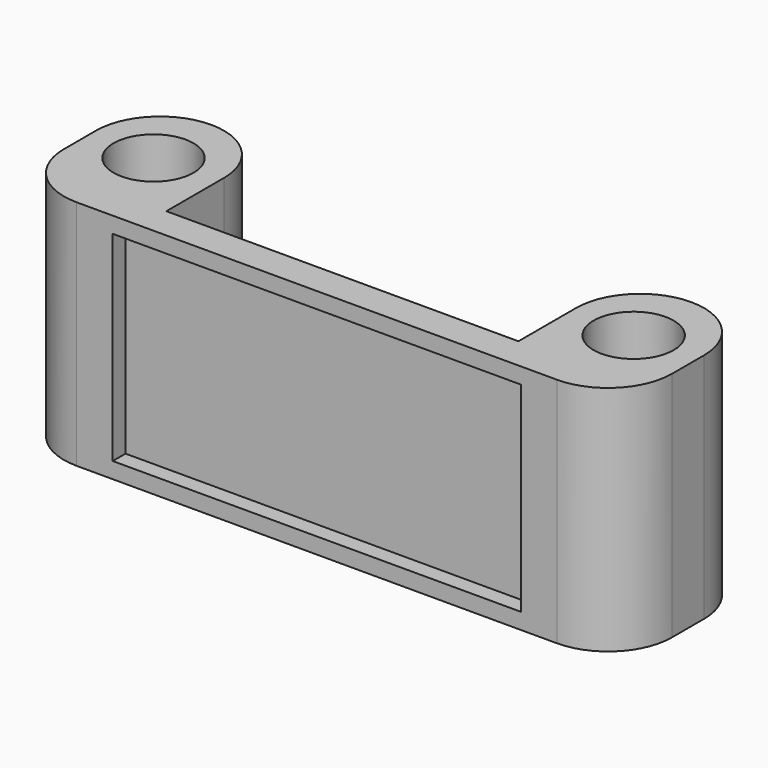
from build123d import *

# Parameters (mm, degrees)
F0_W     = 38
F0_H     = 14.5
F1_DEPTH = 2
F2_W     = 25.5
F2_H     = 12.5
F3_DEPTH = 1
F4_W     = 8
F4_H     = 14.5
F5_DEPTH = 8.5
F6_R     = 2.5
F7_DEPTH = 25
F9_DEPTH = 5
F10_R    = 3.99999


# Not quite as in the source:
# - a fillet or chamfer is up to 0.001 mm smaller than in the source, because OpenCascade refuses the exact size


with BuildPart() as f1:
    # F0 (on Front) → F1 (new body)
    with BuildSketch(Plane.XZ):
        Rectangle(F0_W, F0_H)
    extrude(amount=F1_DEPTH)

    # F2 (on face) → F3 (cut)
    with BuildSketch(Plane.XZ.offset(2)):
        Rectangle(F2_W, F2_H)
    extrude(amount=-F3_DEPTH, mode=Mode.SUBTRACT)

    # F4 (on face) → F5 (join)
    with BuildSketch(Plane(origin=(0, 0, 0), x_dir=(-1, 0, 0), z_dir=(0, 1, 0))):
        with Locations((15, 0)):
            Rectangle(F4_W, F4_H)
        with Locations((-15, 0)):
            Rectangle(F4_W, F4_H)
    extrude(amount=F5_DEPTH)

    # F6 (on face) → F7 (cut)
    with BuildSketch(Plane.XY.offset(7.25)):
        with Locations((-15, 4)):
            Circle(F6_R)
        with Locations((15, 4)):
            Circle(F6_R)
    extrude(amount=-F7_DEPTH, mode=Mode.SUBTRACT)

    # F8 (on face) → F9 (cut)
    with BuildSketch(Plane(origin=(0, 0, -7.25), x_dir=(1, 0, 0), z_dir=(0, 0, -1))):
        Polygon((-15, -7.6661742094), (-11.825, -5.8330871047), (-11.825, -2.1669128953), (-15, -0.3338257906), (-18.175, -2.1669128953), (-18.175, -5.8330871047), align=None)
        Polygon((15, -7.6661742094), (18.175, -5.8330871047), (18.175, -2.1669128953), (15, -0.3338257906), (11.825, -2.1669128953), (11.825, -5.8330871047), align=None)
    extrude(amount=-F9_DEPTH, mode=Mode.SUBTRACT)

    # F10 (radius 4 in the source; OpenCascade refuses exactly that, so slightly less here)
    f10_edges = [f1.edges().sort_by_distance(p)[0] for p in [
        (-19, -2, 0),
        (-19, 8.5, 0),
        (11, 8.5, 0),
        (19, -2, 0),
        (-11, 8.5, 0),
        (19, 8.5, 0),
    ]]
    fillet(f10_edges, radius=F10_R)


solid = f1.part
